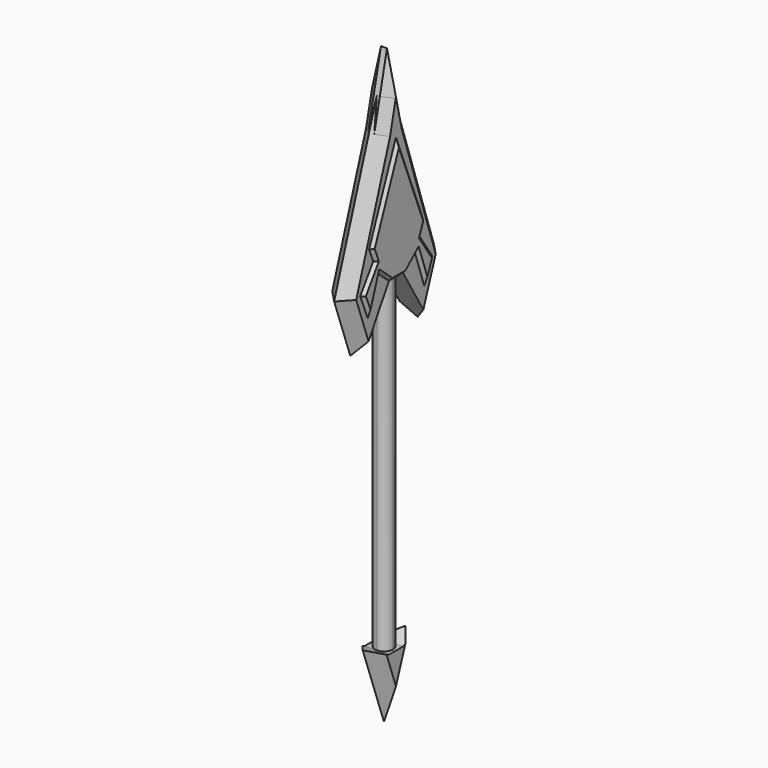
from build123d import *

# Parameters (mm, degrees)
F1_DEPTH     = 3
F2_DEPTH     = 3
F4_DEPTH     = 4
F5_DEPTH     = 4
F6_T1_DEPTH  = 40.486982059
F6_T3_DEPTH  = 40.486982059
F6_T8_DEPTH  = 76.9380455506
F6_T13_DEPTH = 76.9380455506
F6_T18_DEPTH = 76.9380455506
F6_T23_DEPTH = 76.9380455506
F6_T28_DEPTH = 26.5734639037
F6_T35_DEPTH = 26.5734639037
F7_SIZE      = 3
F8_T4_DEPTH  = 125
F8_T10_DEPTH = 125
F8_T16_DEPTH = 125
F8_T22_DEPTH = 125
F9_DEPTH     = 5
F10_DEPTH    = 5
F11_SIZE     = 0.99999
F12_DEPTH    = 4
F13_DEPTH    = 4
F14_SIZE     = 3.99999


# Not quite as in the source:
# - a fillet or chamfer that OpenCascade refuses, or shapes differently, is made with other operations: its cross-section is extruded or revolved along the edge and cut away or added
# - a fillet or chamfer is up to 0.001 mm smaller than in the source, because OpenCascade refuses the exact size


with BuildPart() as f1:
    # F0 (on Right) → F1 (new body)
    with BuildSketch(Plane.YZ):
        Polygon((-3, 55), (-3, 0), (-3, -55), (3, -55), (3, 0), (3, 55), align=None)
    extrude(amount=F1_DEPTH)

    # F0 (on Right) → F2 (join)
    with BuildSketch(Plane.YZ):
        Polygon((-3, 55), (-3, 0), (-3, -55), (3, -55), (3, 0), (3, 55), align=None)
    extrude(amount=-F2_DEPTH)

    # F0 (on Right) → F4 (join)
    with BuildSketch(Plane.YZ):
        Polygon((-14.1003550962, 36.2719446421), (-3, 55), (3, 55), (14.1003550962, 36.2719446421), (20.8685267717, 55), (3, 108.4572896361), (0, 121.4577183127), (-3, 108.4572896361), (-20.8685267717, 55), align=None)
    extrude(amount=F4_DEPTH)

    # F3 (on face) + F0 (on Right) → F5 (join)
    with BuildSketch(Plane.YZ):
        Polygon((-7.805341389, 59.3111515045), (-3.0717977788, 55.1912151277), (3.0717977788, 55.1912151277), (7.805341389, 59.3111515045), (9.517685743, 63.5261535645), (11.2300300971, 67.7411556244), (0, 96.2772667408), (-11.2300300971, 67.7411556244), (-9.517685743, 63.5261535645), align=None)
        Polygon((9.517685743, 63.5261535645), (7.805341389, 59.3111515045), (11.814879576, 47.7191654262), (14.9534028023, 55.4447621107), align=None)
    with BuildSketch(Plane.YZ):
        Polygon((-14.1003550962, 36.2719446421), (-3, 55), (3, 55), (14.1003550962, 36.2719446421), (20.8685267717, 55), (3, 108.4572896361), (0, 121.4577183127), (-3, 108.4572896361), (-20.8685267717, 55), align=None)
    extrude(amount=-F5_DEPTH)

    # F6: chamfer of 4 on 10 edges, made by hand

    # F6_s2 → F6_t1 (cut)
    with BuildSketch(Plane(origin=(0, -23.4873916457, 64.9914322573), x_dir=(1, 0, 0), z_dir=(0, 0.3398782487, -0.9404694445))):
        Polygon((0, 0.932908104), (4, -3.067091896), (4, 0.932908104), align=None)
        Polygon((-4, -3.067091896), (0, 0.932908104), (-4, 0.932908104), align=None)
    extrude(amount=F6_T1_DEPTH, mode=Mode.SUBTRACT)

    # F6_s4 → F6_t3 (cut)
    with BuildSketch(Plane(origin=(0, 9.7267470895, 26.9146627299), x_dir=(1, 0, 0), z_dir=(0, 0.3398782487, 0.9404694445))):
        Polygon((4, -3.067091896), (0, 0.932908104), (4, 0.932908104), align=None)
        Polygon((-4, -3.067091896), (0, 0.932908104), (-4, 0.932908104), align=None)
    extrude(amount=F6_T3_DEPTH, mode=Mode.SUBTRACT)


with BuildPart() as f6_tool6:
    # F6_s7 → F6_t8 (new body)
    with BuildSketch(Plane(origin=(0, -11.1782341891, 33.4419345425), x_dir=(1, 0, 0), z_dir=(0, -0.3170169324, 0.9484198778))):
        Polygon((4, 33.2280568939), (0, 37.2280568939), (4, 37.2280568939), align=None)
    extrude(amount=F6_T8_DEPTH)

    split(bisect_by=Plane(origin=(0, 26.6107337931, 6.1407360761), x_dir=(1, 0, 0), z_dir=(0, 0.9743928202, 0.224852467)), keep=Keep.TOP)


with BuildPart() as f1_1:
    add(f1.part)

    # F6_t5: cut F6_tool6
    add(f6_tool6.part, mode=Mode.SUBTRACT)


with BuildPart() as f6_tool11:
    # F6_s12 → F6_t13 (new body)
    with BuildSketch(Plane(origin=(0, 35.5688973771, 106.4115062996), x_dir=(1, 0, 0), z_dir=(0, -0.3170169324, -0.9484198778))):
        Polygon((4, 33.2280568939), (0, 37.2280568939), (4, 37.2280568939), align=None)
    extrude(amount=F6_T13_DEPTH)

    split(bisect_by=Plane(origin=(0, -26.6107337931, 6.1407360761), x_dir=(1, 0, 0), z_dir=(0, -0.9743928202, 0.224852467)), keep=Keep.TOP)


with BuildPart() as f1_2:
    add(f1_1.part)

    # F6_t10: cut F6_tool11
    add(f6_tool11.part, mode=Mode.SUBTRACT)


with BuildPart() as f6_tool16:
    # F6_s17 → F6_t18 (new body)
    with BuildSketch(Plane(origin=(0, 35.5688973771, 106.4115062996), x_dir=(1, 0, 0), z_dir=(0, -0.3170169324, -0.9484198778))):
        Polygon((-4, 33.2280568939), (0, 37.2280568939), (-4, 37.2280568939), align=None)
    extrude(amount=F6_T18_DEPTH)

    split(bisect_by=Plane(origin=(0, -26.6107337931, 6.1407360761), x_dir=(1, 0, 0), z_dir=(0, -0.9743928202, 0.224852467)), keep=Keep.TOP)


with BuildPart() as f1_3:
    add(f1_2.part)

    # F6_t15: cut F6_tool16
    add(f6_tool16.part, mode=Mode.SUBTRACT)


with BuildPart() as f6_tool21:
    # F6_s22 → F6_t23 (new body)
    with BuildSketch(Plane(origin=(0, -11.1782341891, 33.4419345425), x_dir=(1, 0, 0), z_dir=(0, -0.3170169324, 0.9484198778))):
        Polygon((-4, 33.2280568939), (0, 37.2280568939), (-4, 37.2280568939), align=None)
    extrude(amount=F6_T23_DEPTH)

    split(bisect_by=Plane(origin=(0, 26.6107337931, 6.1407360761), x_dir=(1, 0, 0), z_dir=(0, 0.9743928202, 0.224852467)), keep=Keep.TOP)


with BuildPart() as f1_4:
    add(f1_3.part)

    # F6_t20: cut F6_tool21
    add(f6_tool21.part, mode=Mode.SUBTRACT)


with BuildPart() as f6_tool26:
    # F6_s27 → F6_t28 (new body)
    with BuildSketch(Plane.XZ.offset(13.2867319519)):
        Polygon((0, 55), (-4, 59), (-4, 55), align=None)
    extrude(amount=-F6_T28_DEPTH)

    split(bisect_by=Plane.YZ.offset(-3), keep=Keep.BOTTOM)

    split(bisect_by=Plane(origin=(0, 26.3442442024, 15.6145664778), x_dir=(1, 0, 0), z_dir=(0, -0.8602462388, -0.5098788176)), keep=Keep.TOP)

    split(bisect_by=Plane(origin=(0, -26.3442442024, 15.6145664778), x_dir=(1, 0, 0), z_dir=(0, 0.8602462388, -0.5098788176)), keep=Keep.TOP)


with BuildPart() as f1_5:
    add(f1_4.part)

    # F6_t25: cut F6_tool26
    add(f6_tool26.part, mode=Mode.SUBTRACT)


with BuildPart() as f6_tool33:
    # F6_s34 → F6_t35 (new body)
    with BuildSketch(Plane.XZ.offset(13.2867319519)):
        Polygon((4, 59), (0, 55), (4, 55), align=None)
    extrude(amount=-F6_T35_DEPTH)

    split(bisect_by=Plane.YZ.offset(3), keep=Keep.TOP)

    split(bisect_by=Plane(origin=(0, 26.3442442024, 15.6145664778), x_dir=(1, 0, 0), z_dir=(0, -0.8602462388, -0.5098788176)), keep=Keep.TOP)

    split(bisect_by=Plane(origin=(0, -26.3442442024, 15.6145664778), x_dir=(1, 0, 0), z_dir=(0, 0.8602462388, -0.5098788176)), keep=Keep.TOP)


with BuildPart() as f1_6:
    add(f1_5.part)

    # F6_t32: cut F6_tool33
    add(f6_tool33.part, mode=Mode.SUBTRACT)

    # F7
    f7_edges = [f1_6.edges().sort_by_distance(p)[0] for p in [
        (4, 6.201839, 94.582196),
        (4, -6.201839, 94.582196),
        (-4, -6.201839, 94.582196),
        (-4, 6.201839, 94.582196),
    ]]
    chamfer(f7_edges, length=F7_SIZE)

    # F8: fillet of radius 3 on 4 edges, made by hand


with BuildPart() as f8_tool2:
    # F8_s3 → F8_t4 (new body)
    with BuildSketch(Plane.XY.offset(62.5)):
        with BuildLine():
            ThreePointArc((0, -3), (-2.1213203436, -2.1213203436), (-3, 0))
            Line((-3, 0), (-3, -3))
            Line((-3, -3), (0, -3))
        make_face()
    extrude(amount=-F8_T4_DEPTH)

    split(bisect_by=Plane(origin=(0, -26.3442442024, 15.6145664778), x_dir=(1, 0, 0), z_dir=(0, 0.8602462388, -0.5098788176)), keep=Keep.TOP)

    split(bisect_by=Plane(origin=(27.5, 0, 27.5), x_dir=(0, 1, 0), z_dir=(-0.7071067812, 0, -0.7071067812)), keep=Keep.TOP)


with BuildPart() as f1_7:
    add(f1_6.part)

    # F8_t1: cut F8_tool2
    add(f8_tool2.part, mode=Mode.SUBTRACT)


with BuildPart() as f8_tool8:
    # F8_s9 → F8_t10 (new body)
    with BuildSketch(Plane.XY.offset(-62.5)):
        with BuildLine():
            ThreePointArc((-3, 0), (-2.1213203436, 2.1213203436), (0, 3))
            Line((0, 3), (-3, 3))
            Line((-3, 3), (-3, 0))
        make_face()
    extrude(amount=F8_T10_DEPTH)

    split(bisect_by=Plane(origin=(27.5, 0, 27.5), x_dir=(0, 1, 0), z_dir=(-0.7071067812, 0, -0.7071067812)), keep=Keep.TOP)

    split(bisect_by=Plane(origin=(0, 26.3442442024, 15.6145664778), x_dir=(1, 0, 0), z_dir=(0, -0.8602462388, -0.5098788176)), keep=Keep.TOP)


with BuildPart() as f1_8:
    add(f1_7.part)

    # F8_t7: cut F8_tool8
    add(f8_tool8.part, mode=Mode.SUBTRACT)


with BuildPart() as f8_tool14:
    # F8_s15 → F8_t16 (new body)
    with BuildSketch(Plane.XY.offset(62.5)):
        with BuildLine():
            ThreePointArc((3, 0), (2.1213203436, 2.1213203436), (0, 3))
            Line((0, 3), (3, 3))
            Line((3, 3), (3, 0))
        make_face()
    extrude(amount=-F8_T16_DEPTH)

    split(bisect_by=Plane(origin=(0, 26.3442442024, 15.6145664778), x_dir=(1, 0, 0), z_dir=(0, -0.8602462388, -0.5098788176)), keep=Keep.TOP)

    split(bisect_by=Plane(origin=(-27.5, 0, 27.5), x_dir=(0, 1, 0), z_dir=(0.7071067812, 0, -0.7071067812)), keep=Keep.TOP)


with BuildPart() as f1_9:
    add(f1_8.part)

    # F8_t13: cut F8_tool14
    add(f8_tool14.part, mode=Mode.SUBTRACT)


with BuildPart() as f8_tool20:
    # F8_s21 → F8_t22 (new body)
    with BuildSketch(Plane.XY.offset(-62.5)):
        with BuildLine():
            ThreePointArc((3, 0), (2.1213203436, -2.1213203436), (0, -3))
            Line((0, -3), (3, -3))
            Line((3, -3), (3, 0))
        make_face()
    extrude(amount=F8_T22_DEPTH)

    split(bisect_by=Plane(origin=(0, -26.3442442024, 15.6145664778), x_dir=(1, 0, 0), z_dir=(0, 0.8602462388, -0.5098788176)), keep=Keep.TOP)

    split(bisect_by=Plane(origin=(-27.5, 0, 27.5), x_dir=(0, 1, 0), z_dir=(0.7071067812, 0, -0.7071067812)), keep=Keep.TOP)


with BuildPart() as f1_10:
    add(f1_9.part)

    # F8_t19: cut F8_tool20
    add(f8_tool20.part, mode=Mode.SUBTRACT)

    # F3 (on face) → F9 (join)
    with BuildSketch(Plane.YZ):
        Polygon((-7.805341389, 59.3111515045), (-3.0717977788, 55.1912151277), (3.0717977788, 55.1912151277), (7.805341389, 59.3111515045), (9.517685743, 63.5261535645), (11.2300300971, 67.7411556244), (0, 96.2772667408), (-11.2300300971, 67.7411556244), (-9.517685743, 63.5261535645), align=None)
        Polygon((-11.814879576, 47.7191654262), (-7.805341389, 59.3111515045), (-9.517685743, 63.5261535645), (-14.9534028023, 55.4447621107), align=None)
        Polygon((9.517685743, 63.5261535645), (7.805341389, 59.3111515045), (11.814879576, 47.7191654262), (14.9534028023, 55.4447621107), align=None)
    extrude(amount=F9_DEPTH)

    # F3 (on face) → F10 (join)
    with BuildSketch(Plane.YZ):
        Polygon((-7.805341389, 59.3111515045), (-3.0717977788, 55.1912151277), (3.0717977788, 55.1912151277), (7.805341389, 59.3111515045), (9.517685743, 63.5261535645), (11.2300300971, 67.7411556244), (0, 96.2772667408), (-11.2300300971, 67.7411556244), (-9.517685743, 63.5261535645), align=None)
        Polygon((-11.814879576, 47.7191654262), (-7.805341389, 59.3111515045), (-9.517685743, 63.5261535645), (-14.9534028023, 55.4447621107), align=None)
        Polygon((9.517685743, 63.5261535645), (7.805341389, 59.3111515045), (11.814879576, 47.7191654262), (14.9534028023, 55.4447621107), align=None)
    extrude(amount=-F10_DEPTH)

    # F11 (size 1 in the source; OpenCascade refuses exactly that, so slightly less here)
    f11_edges = [f1_10.edges().sort_by_distance(p)[0] for p in [
        (5, -5.43857, 57.251183),
        (5, 0, 55.191215),
        (5, 5.43857, 57.251183),
        (5, 9.81011, 53.515158),
        (5, 13.384141, 51.581964),
        (5, 12.235544, 59.485458),
        (5, 10.373858, 65.633655),
        (5, 5.615015, 82.009211),
        (5, -5.615015, 82.009211),
        (5, -10.373858, 65.633655),
        (5, -12.235544, 59.485458),
        (5, -13.384141, 51.581964),
        (5, -9.81011, 53.515158),
        (-5, -5.615015, 82.009211),
        (-5, -5.43857, 57.251183),
        (-5, 0, 55.191215),
        (-5, 5.43857, 57.251183),
        (-5, 9.81011, 53.515158),
        (-5, 13.384141, 51.581964),
        (-5, 12.235544, 59.485458),
        (-5, 10.373858, 65.633655),
        (-5, 5.615015, 82.009211),
        (-5, -10.373858, 65.633655),
        (-5, -12.235544, 59.485458),
        (-5, -13.384141, 51.581964),
        (-5, -9.81011, 53.515158),
    ]]
    chamfer(f11_edges, length=F11_SIZE)

    # F0 (on Right) → F12 (join)
    with BuildSketch(Plane.YZ):
        Polygon((3, -55), (-3, -55), (-8.9030144736, -52.6038594544), (0, -77.3145779967), (8.9030144736, -52.6038594544), align=None)
    extrude(amount=F12_DEPTH)

    # F0 (on Right) → F13 (join)
    with BuildSketch(Plane.YZ):
        Polygon((3, -55), (-3, -55), (-8.9030144736, -52.6038594544), (0, -77.3145779967), (8.9030144736, -52.6038594544), align=None)
    extrude(amount=-F13_DEPTH)

    # F14 (size 4 in the source; OpenCascade refuses exactly that, so slightly less here)
    f14_edges = [f1_10.edges().sort_by_distance(p)[0] for p in [
        (-4, -4.451507, -64.959219),
        (-4, 4.451507, -64.959219),
        (4, -4.451507, -64.959219),
        (4, 4.451507, -64.959219),
    ]]
    chamfer(f14_edges, length=F14_SIZE)


solid = f1_10.part
